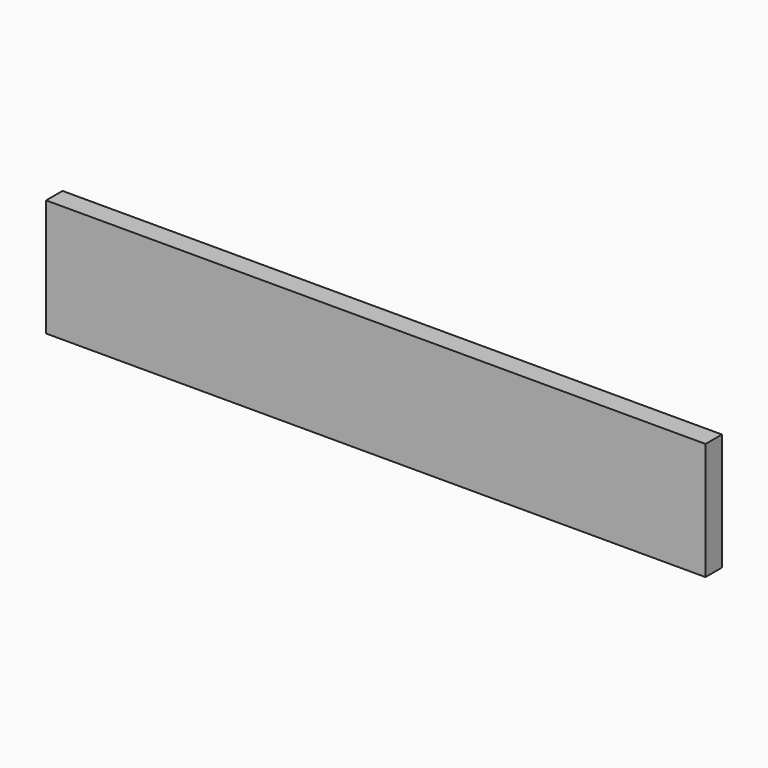
from build123d import *

# Parameters (mm, degrees)
F1_DEPTH = 3.5


# Not quite as in the source:
# - ends of sketch curves that miss each other by under 0.0002 mm in the source are joined


with BuildPart() as f1:
    # F0 (on Front) → F1 (new body, symmetric)
    with BuildSketch(Plane.XZ):
        Polygon((112.5, 20), (-4.327e-06, 20), (-112.5, 20), (-112.5, 0), (-112.5, -20), (4.327e-06, -20), (112.5, -20), (112.5, 0), align=None)
    extrude(amount=F1_DEPTH, both=True)


solid = f1.part
